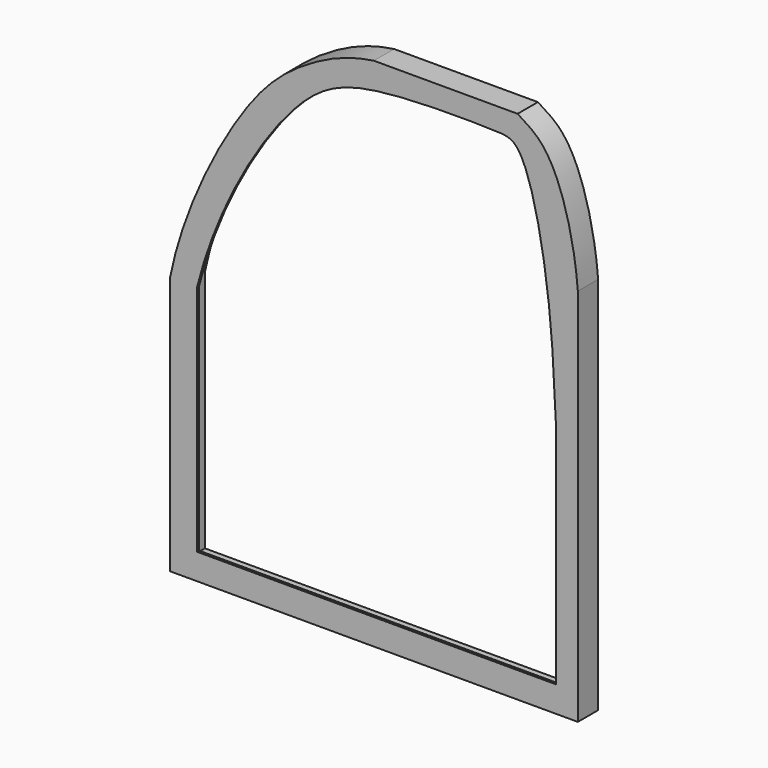
from build123d import *

# Parameters (mm, degrees)
F1_DEPTH = 5
F2_DEPTH = 0.5


with BuildPart() as f1:
    # F0 (on Front) → F1 (new body)
    with BuildSketch(Plane.XZ):
        with BuildLine():
            Line((21.9498877709, 46.5069999899), (-6.3801594079, 46.5069999899))
            add(Edge.make_bspline(
                [(-46.5855710208, -4.3176412582), (-44.0025745855, 8.8650835819), (-32.3669471438, 31.5826223404), (-20.8450996019, 41.430559805), (-11.9788710798, 45.7277535437), (-6.3801594079, 46.5069999899)],
                knots=[0, 0, 0, 0, 0.4471722481, 0.7226417186, 1, 1, 1, 1], degree=3))
            Line((-46.5855710208, -4.3176412582), (-46.5855710208, -55.1422825063))
            Line((-46.5855710208, -55.1422825063), (33.8252522051, -55.1422825063))
            Line((33.8252522051, -55.1422825063), (33.8252522051, 3.3716567512))
            add(Edge.make_bspline(
                [(33.8252522051, 3.4864664458), (33.8224510146, 3.4189701607), (33.823496077, 3.4012213221), (33.8252522051, 3.3716567512)],
                knots=[0.9714616128, 0.9714616128, 0.9714616128, 0.9714616128, 1, 1, 1, 1], degree=3))
            Line((33.8252522051, 3.4864664458), (33.8252522051, 19.6025110781))
            add(Edge.make_bspline(
                [(21.9498877709, 46.5069999899), (23.8964492564, 45.3404017708), (29.3341911452, 42.1357952335), (33.1026848595, 28.5809846581), (33.8252522051, 19.6025110781)],
                knots=[0, 0, 0, 0, 0.2303722913, 0.6333427683, 0.6333427683, 0.6333427683, 0.6333427683], degree=3))
        make_face()
        with BuildLine():
            Line((31.6210500896, -52.260261029), (-43.6766035855, -52.260261029))
            Line((-43.6766035855, -52.260261029), (-43.6766035855, -4.3176412582))
            add(Edge.make_bspline(
                [(-43.6766035855, -4.3176412582), (-41.0383021138, 9.0666906176), (-27.9398807539, 30.9156219348), (-18.7479844266, 41.3390835094), (-7.0085331076, 43.5985571671), (-2.215007715, 43.8020735184), (21.2993443911, 44.9657713637), (26.0800513958, 41.7197839808), (31.3102526714, 18.3624746495), (31.5930695379, 3.1075431018), (31.6210500896, -4.3176412582)],
                knots=[0, 0, 0, 0, 0.1942047864, 0.3092342936, 0.40822929, 0.4837495286, 0.6306580628, 0.7017097882, 0.8479049191, 1, 1, 1, 1], degree=3))
            Line((31.6210500896, -4.3176412582), (31.6210500896, -52.260261029))
        make_face(mode=Mode.SUBTRACT)
        with BuildLine():
            Line((33.8252522051, 3.3716567512), (33.8252522051, 3.4864664458))
            add(Edge.make_bspline(
                [(33.8252522051, 3.4864664458), (33.8224510146, 3.4189701607), (33.823496077, 3.4012213221), (33.8252522051, 3.3716567512)],
                knots=[0.9714616128, 0.9714616128, 0.9714616128, 0.9714616128, 1, 1, 1, 1], degree=3))
        make_face()
    extrude(amount=-F1_DEPTH)

    # F0 (on Front) → F2 (join)
    with BuildSketch(Plane.XZ):
        with BuildLine():
            Line((-43.6766035855, -4.3176412582), (-43.6766035855, -52.260261029))
            Line((-43.6766035855, -52.260261029), (31.6210500896, -52.260261029))
            Line((31.6210500896, -52.260261029), (31.6210500896, -4.3176412582))
            add(Edge.make_bspline(
                [(-43.6766035855, -4.3176412582), (-41.0383021138, 9.0666906176), (-27.9398807539, 30.9156219348), (-18.7479844266, 41.3390835094), (-7.0085331076, 43.5985571671), (-2.215007715, 43.8020735184), (21.2993443911, 44.9657713637), (26.0800513958, 41.7197839808), (31.3102526714, 18.3624746495), (31.5930695379, 3.1075431018), (31.6210500896, -4.3176412582)],
                knots=[0, 0, 0, 0, 0.1942047864, 0.3092342936, 0.40822929, 0.4837495286, 0.6306580628, 0.7017097882, 0.8479049191, 1, 1, 1, 1], degree=3))
        make_face()
        with BuildLine():
            Line((29.4725894928, -50.028309226), (-41.2763357162, -50.028309226))
            Line((-41.2763357162, -50.028309226), (-41.2763357162, -4.3176412582))
            add(Edge.make_bspline(
                [(29.4725894928, -4.3176412582), (29.1241496967, 2.9787885737), (28.5454511929, 18.1687452905), (23.4164160844, 41.9172876242), (16.665337298, 42.2003372333), (-7.4096989865, 42.5160002908), (-22.9090094529, 36.1722681351), (-37.4855825891, 11.2133633357), (-41.2763357162, -4.3176412582)],
                knots=[0, 0, 0, 0, 0.1793175303, 0.3494515687, 0.4340680096, 0.6090858367, 0.7583926872, 1, 1, 1, 1], degree=3))
            Line((29.4725894928, -4.3176412582), (29.4725894928, -50.028309226))
        make_face(mode=Mode.SUBTRACT)
    extrude(amount=-F2_DEPTH)


solid = f1.part
